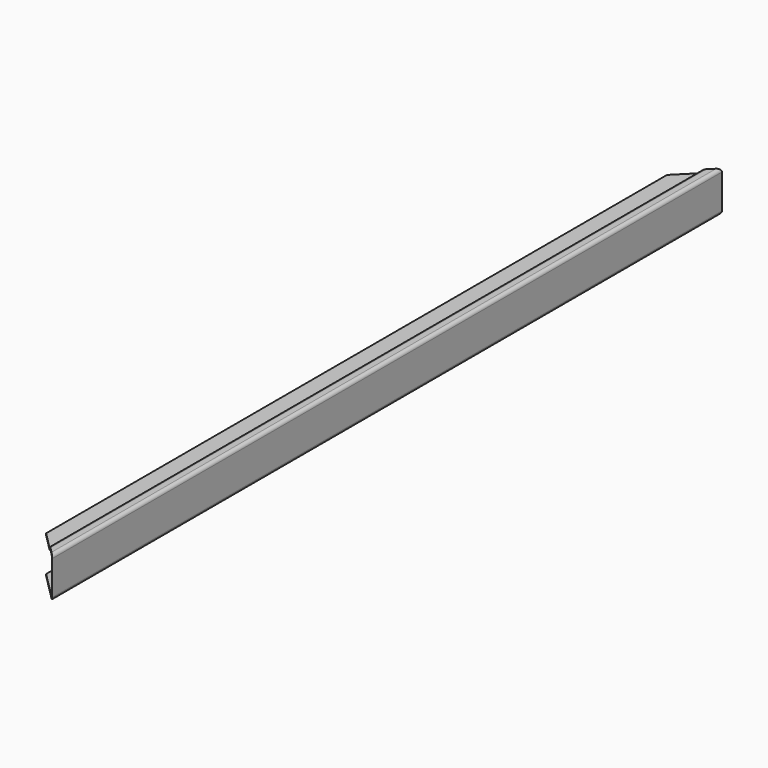
from build123d import *

# Parameters (mm, degrees)
F1_DEPTH                = 2059
F4_W                    = 350
F4_H                    = 150
F5_DEPTH                = 150
F15_W                   = 255.14793396
F15_H                   = 122.3266422749
F16_DEPTH               = 200
DRAFT_F16_DRAFTED_ANGLE = -3


# Not quite as in the source:
# - an extrude with a draft is written as a straight extrude whose walls are then drafted


with BuildPart() as f1:
    # F0 (on Front) → F1 (new body)
    with BuildSketch(Plane.XZ):
        with BuildLine():
            ThreePointArc((-37.5, -42), (-35.1568542495, -47.6568542495), (-29.5, -50))
            Line((-29.5, -50), (37.5, -50))
            Line((37.5, -50), (37.5, -46))
            Line((37.5, -46), (-29.5, -46))
            ThreePointArc((-29.5, -46), (-32.3284271247, -44.8284271247), (-33.5, -42))
            Line((-33.5, -42), (-33.5, 42))
            ThreePointArc((-33.5, 42), (-32.3284271247, 44.8284271247), (-29.5, 46))
            Line((-29.5, 46), (-16.2304612652, 46))
            ThreePointArc((-16.2304612652, 46), (-14.5399882183, 45.6252311481), (-13.1662834928, 44.5711504387))
            Line((-13.1662834928, 44.5711504387), (-10.0503278629, 40.8576991225))
            ThreePointArc((-10.0503278629, 40.8576991225), (-7.3029184119, 38.7495377037), (-3.921972318, 38))
            Line((-3.921972318, 38), (37.5, 38))
            Line((37.5, 38), (37.5, 42))
            Line((37.5, 42), (-3.921972318, 42))
            ThreePointArc((-3.921972318, 42), (-5.6124453649, 42.3747688519), (-6.9861500904, 43.4288495613))
            Line((-6.9861500904, 43.4288495613), (-10.1021057203, 47.1423008775))
            ThreePointArc((-10.1021057203, 47.1423008775), (-12.8495151713, 49.2504622963), (-16.2304612652, 50))
            Line((-16.2304612652, 50), (-29.5, 50))
            ThreePointArc((-29.5, 50), (-35.1568542495, 47.6568542495), (-37.5, 42))
            Line((-37.5, 42), (-37.5, -42))
        make_face()
    extrude(amount=-F1_DEPTH)

    # F4 (on face) → F5 (cut)
    with BuildSketch(Plane(origin=(-18.75, 18.75, 0), x_dir=(0.7071067812, 0.7071067812, 0), z_dir=(0.7071067812, -0.7071067812, 0))):
        Rectangle(F4_W, F4_H)
    extrude(amount=F5_DEPTH, mode=Mode.SUBTRACT)


with BuildPart() as f7_1:
    # F7: instance of F1
    add(f1.part.mirror(Plane.YZ.offset(200)))

    # F8: F1 across plane
    add(f1.part.mirror(Plane.YZ.offset(200)))


with BuildPart() as f10_1:
    # F10: instance of F1
    add(f1.part.mirror(Plane.YZ.offset(700)))


with BuildPart() as f16_drafted:
    # F15 (on face) → F16 (new body)
    with BuildSketch(Plane(origin=(-310.75, 310.75, 0), x_dir=(0.7071067812, 0.7071067812, 0), z_dir=(0.7071067812, -0.7071067812, 0))):
        with Locations((2394.6449756622, 11.1766308546)):
            Rectangle(F15_W, F15_H)
    extrude(amount=-F16_DEPTH)

    # draft_F16_drafted
    draft_f16_drafted_walls = [f16_drafted.faces().sort_by_distance(p)[0] for p in [
        (1288.2387966669, 2098.3006049833, -49.9866902828),
        (1378.4472138213, 2188.5090221377, 11.1766308546),
        (1288.2387966669, 2098.3006049833, 72.339951992),
        (1198.0303795124, 2008.0921878289, 11.1766308546),
    ]]
    draft(draft_f16_drafted_walls, neutral_plane=Plane(origin=(-310.75, 310.75, 0), x_dir=(0.7071067812, 0.7071067812, 0), z_dir=(-0.7071067812, 0.7071067812, 0)), angle=DRAFT_F16_DRAFTED_ANGLE)


with BuildPart() as f10_1_1:
    add(f10_1.part)

    # join_F16_drafted: cut F16_drafted
    add(f16_drafted.part, mode=Mode.SUBTRACT)


solid = f10_1_1.part
